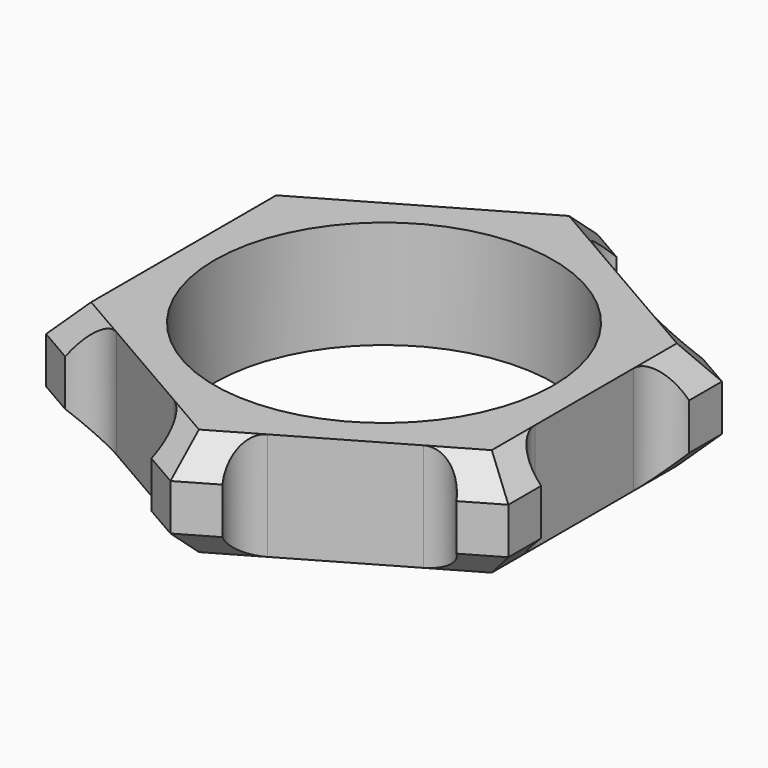
from build123d import *

# Parameters (mm, degrees)
F0_R            = 11
F1_DEPTH        = 7
F2_SIZE         = 2
F4_DEPTH        = 25
F4_COPIES_COUNT = 6


# Not quite as in the source:
# - a pattern or mirror of a feature is missing from the dataset's text; its kind, count and spacing are read off the source's solid


with BuildPart() as f1:
    # F0 (on Top) → F1 (new body)
    with BuildSketch(Plane.XY):
        Polygon((15, -8.6602540378), (15, 8.6602540378), (0, 17.3205080757), (-15, 8.6602540378), (-15, -8.6602540378), (0, -17.3205080757), align=None)
        Circle(F0_R, mode=Mode.SUBTRACT)
    extrude(amount=F1_DEPTH)

    # F2
    f2_edges = [f1.edges().sort_by_distance(p)[0] for p in [
        (-15, 0, 7),
        (-7.5, 12.990381, 7),
        (7.5, 12.990381, 7),
        (15, 0, 7),
        (7.5, -12.990381, 7),
        (-7.5, -12.990381, 7),
        (-15, 0, 0),
        (-7.5, 12.990381, 0),
        (7.5, 12.990381, 0),
        (15, 0, 0),
        (7.5, -12.990381, 0),
        (-7.5, -12.990381, 0),
    ]]
    chamfer(f2_edges, length=F2_SIZE)

    # F3 (on Top) → F4 (cut)
    with BuildSketch(Plane.XY):
        Polygon((17, 6), (15, 6), (15, -6), (17, -6), (17, -4), (17, 4), align=None)
        with BuildLine():
            Line((15, -6), (15, 6))
            ThreePointArc((15, 6), (13.5857864376, 5.4142135624), (13, 4))
            Line((13, 4), (13, -4))
            ThreePointArc((13, -4), (13.5857864376, -5.4142135624), (15, -6))
        make_face()
    f4 = extrude(amount=F4_DEPTH, mode=Mode.SUBTRACT)

    # F4_copies: F4 ×6 about axis
    f4_copies_axis = Axis((0, 0, 0), (0, 0, 1))
    for i in range(1, F4_COPIES_COUNT):
        add(f4.rotate(f4_copies_axis, i * 360 / F4_COPIES_COUNT), mode=Mode.SUBTRACT)


solid = f1.part
